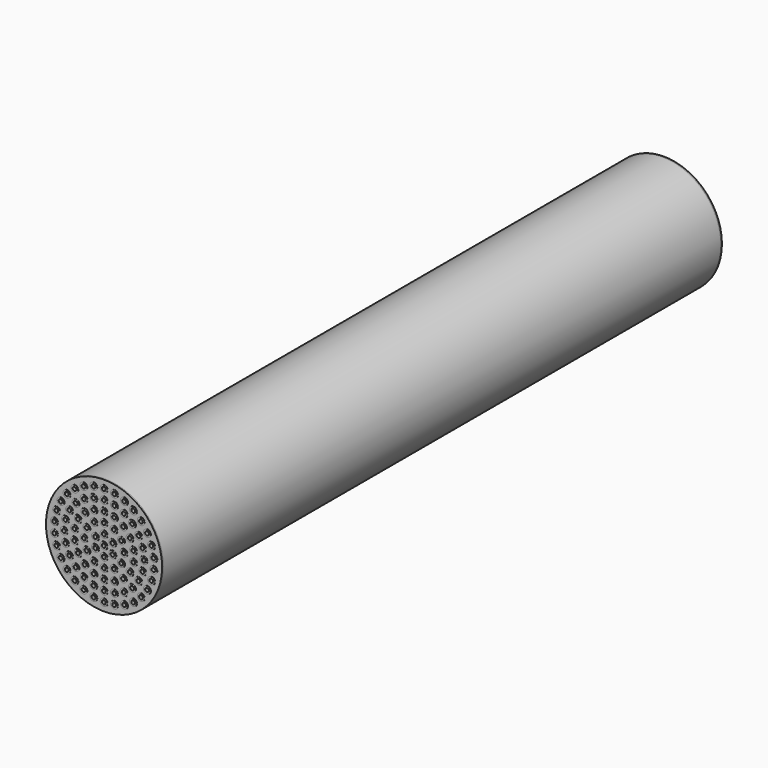
from build123d import *

# Parameters (mm, degrees)
F0_R          = 50.8
F0_R_2        = 49.276
F1_DEPTH      = 609.6
F0_R_3        = 3.175
F2_DEPTH      = 611.124
F2_DEPTH_BACK = 1.524
F3_T          = -1.524
F4_START      = 609.6
F4_DEPTH      = 1.27
F5_DEPTH      = 1.27


# Not quite as in the source:
# - a shell that OpenCascade refuses in one call is made with other operations: the cavity is built on its own and cut out


with BuildPart() as f1:
    # F0 (on Front) → F1 (new body)
    with BuildSketch(Plane.XZ):
        Circle(F0_R)
        Circle(F0_R_2, mode=Mode.SUBTRACT)
    extrude(amount=F1_DEPTH)


with BuildPart() as f2:
    # F0 (on Front) → F2 (new body, two sides)
    with BuildSketch(Plane.XZ) as f2_sk:
        with Locations((32.4429162872, 29.2117330339)):
            Circle(F0_R_3)
        with Locations((22.6844529204, -13.096875)):
            Circle(F0_R_3)
        with Locations((-9.0392551502, -33.7349594831)):
            Circle(F0_R_3)
        with Locations((-17.4625, -30.2459372272)):
            Circle(F0_R_3)
        with Locations((-8.9587901292, 24.6140735857)):
            Circle(F0_R_3)
        with Locations((-37.807421534, -21.828125)):
            Circle(F0_R_3)
        with Locations((-32.4429162872, -29.2117330339)):
            Circle(F0_R_3)
        with Locations((-30.2459372272, -17.4625)):
            Circle(F0_R_3)
        with Locations((-22.6844529204, 13.096875)):
            Circle(F0_R_3)
        with Locations((17.7565965743, -39.8819688852)):
            Circle(F0_R_3)
        with Locations((-9.0766447523, 42.7022561945)):
            Circle(F0_R_3)
        with Locations((25.7958080805, -4.5484969538)):
            Circle(F0_R_3)
        with Locations((0, -34.925)):
            Circle(F0_R_3)
        with Locations((-9.0766447523, -42.7022561945)):
            Circle(F0_R_3)
        with Locations((17.7565965743, 39.8819688852)):
            Circle(F0_R_3)
        with Locations((-25.6604999204, -35.3186481607)):
            Circle(F0_R_3)
        with Locations((-15.1229686136, -8.73125)):
            Circle(F0_R_3)
        with Locations((-41.5195610395, 13.4905231607)):
            Circle(F0_R_3)
        with Locations((9.0392551502, -33.7349594831)):
            Circle(F0_R_3)
        with Locations((-16.8370179512, -20.0655766319)):
            Circle(F0_R_3)
        with Locations((8.9587901292, -24.6140735857)):
            Circle(F0_R_3)
        with Locations((37.807421534, -21.828125)):
            Circle(F0_R_3)
        with Locations((16.8370179512, -20.0655766319)):
            Circle(F0_R_3)
        with Locations((25.7958080805, 4.5484969538)):
            Circle(F0_R_3)
        with Locations((43.4170964947, 4.5633207245)):
            Circle(F0_R_3)
        with Locations((-24.6957043329, -24.6957043329)):
            Circle(F0_R_3)
        with Locations((-33.7349594831, -9.0392551502)):
            Circle(F0_R_3)
        with Locations((-8.9587901292, -24.6140735857)):
            Circle(F0_R_3)
        with Locations((16.8370179512, 20.0655766319)):
            Circle(F0_R_3)
        with Locations((-15.1229686136, 8.73125)):
            Circle(F0_R_3)
        with Locations((33.7349594831, -9.0392551502)):
            Circle(F0_R_3)
        with Locations((9.0766447523, 42.7022561945)):
            Circle(F0_R_3)
        with Locations((0, 8.73125)):
            Circle(F0_R_3)
        with Locations((0, 34.925)):
            Circle(F0_R_3)
        with Locations((0, 43.65625)):
            Circle(F0_R_3)
        with Locations((-7.5614843068, -4.365625)):
            Circle(F0_R_3)
        with Locations((-7.5614843068, 4.365625)):
            Circle(F0_R_3)
        with Locations((7.5614843068, 4.365625)):
            Circle(F0_R_3)
        with Locations((-8.73125, 15.1229686136)):
            Circle(F0_R_3)
        with Locations((0, -17.4625)):
            Circle(F0_R_3)
        with Locations((37.807421534, 21.828125)):
            Circle(F0_R_3)
        with Locations((30.2459372272, -17.4625)):
            Circle(F0_R_3)
        with Locations((34.925, 0)):
            Circle(F0_R_3)
        with Locations((24.6957043329, 24.6957043329)):
            Circle(F0_R_3)
        with Locations((25.6604999204, 35.3186481607)):
            Circle(F0_R_3)
        with Locations((15.1229686136, -8.73125)):
            Circle(F0_R_3)
        with Locations((41.5195610395, -13.4905231607)):
            Circle(F0_R_3)
        with Locations((-37.807421534, 21.828125)):
            Circle(F0_R_3)
        with Locations((-43.4170964947, -4.5633207245)):
            Circle(F0_R_3)
        with Locations((41.5195610395, 13.4905231607)):
            Circle(F0_R_3)
        with Locations((17.4625, 0)):
            Circle(F0_R_3)
        with Locations((43.4170964947, -4.5633207245)):
            Circle(F0_R_3)
        with Locations((17.4625, 30.2459372272)):
            Circle(F0_R_3)
        with Locations((-34.925, 0)):
            Circle(F0_R_3)
        with Locations((-25.7958080805, -4.5484969538)):
            Circle(F0_R_3)
        with Locations((0, -26.19375)):
            Circle(F0_R_3)
        with Locations((15.1229686136, 8.73125)):
            Circle(F0_R_3)
        with Locations((-17.7565965743, -39.8819688852)):
            Circle(F0_R_3)
        with Locations((9.0766447523, -42.7022561945)):
            Circle(F0_R_3)
        with Locations((9.0392551502, 33.7349594831)):
            Circle(F0_R_3)
        with Locations((17.4625, -30.2459372272)):
            Circle(F0_R_3)
        with Locations((22.6844529204, 13.096875)):
            Circle(F0_R_3)
        with Locations((-22.6844529204, -13.096875)):
            Circle(F0_R_3)
        with Locations((-33.7349594831, 9.0392551502)):
            Circle(F0_R_3)
        with Locations((32.4429162872, -29.2117330339)):
            Circle(F0_R_3)
        with Locations((33.7349594831, 9.0392551502)):
            Circle(F0_R_3)
        with Locations((-17.4625, 30.2459372272)):
            Circle(F0_R_3)
        with Locations((-24.6957043329, 24.6957043329)):
            Circle(F0_R_3)
        with Locations((-25.7958080805, 4.5484969538)):
            Circle(F0_R_3)
        with Locations((24.6957043329, -24.6957043329)):
            Circle(F0_R_3)
        with Locations((8.73125, 15.1229686136)):
            Circle(F0_R_3)
        with Locations((-25.6604999204, 35.3186481607)):
            Circle(F0_R_3)
        with Locations((-17.4625, 0)):
            Circle(F0_R_3)
        with Locations((-8.73125, -15.1229686136)):
            Circle(F0_R_3)
        with Locations((25.6604999204, -35.3186481607)):
            Circle(F0_R_3)
        with Locations((-17.7565965743, 39.8819688852)):
            Circle(F0_R_3)
        with Locations((0, -43.65625)):
            Circle(F0_R_3)
        with Locations((30.2459372272, 17.4625)):
            Circle(F0_R_3)
        with Locations((-30.2459372272, 17.4625)):
            Circle(F0_R_3)
        with Locations((8.73125, -15.1229686136)):
            Circle(F0_R_3)
        Circle(F0_R_3)
        with Locations((-43.4170964947, 4.5633207245)):
            Circle(F0_R_3)
        with Locations((0, 26.19375)):
            Circle(F0_R_3)
        with Locations((0, 17.4625)):
            Circle(F0_R_3)
        with Locations((0, -8.73125)):
            Circle(F0_R_3)
        with Locations((-32.4429162872, 29.2117330339)):
            Circle(F0_R_3)
        with Locations((7.5614843068, -4.365625)):
            Circle(F0_R_3)
        with Locations((-9.0392551502, 33.7349594831)):
            Circle(F0_R_3)
        with Locations((8.9587901292, 24.6140735857)):
            Circle(F0_R_3)
        with Locations((-41.5195610395, -13.4905231607)):
            Circle(F0_R_3)
        with Locations((-16.8370179512, 20.0655766319)):
            Circle(F0_R_3)
    extrude(amount=F2_DEPTH)
    extrude(f2_sk.sketch, amount=-F2_DEPTH_BACK)

    # F3: a shell. OpenCascade refuses it in one call, so the cavity is built on its own and cut out:
    # the body offset inwards by the wall thickness, plus a prism from it out through each open face.
    f3_core = offset(f2.part, amount=F3_T, kind=Kind.INTERSECTION, mode=Mode.PRIVATE)
    f3_exits = [f3_core.faces().sort_by_distance(p)[0] for p in [
        (0, -609.6, -43.65625),
        (-9.076645, -609.6, -42.702256),
        (-17.756597, -609.6, -39.881969),
        (-25.6605, -609.6, -35.318648),
        (-32.442916, -609.6, -29.211733),
        (-37.807422, -609.6, -21.828125),
        (-41.519561, -609.6, -13.490523),
        (-43.417096, -609.6, -4.563321),
        (-43.417096, -609.6, 4.563321),
        (-41.519561, -609.6, 13.490523),
        (-37.807422, -609.6, 21.828125),
        (-32.442916, -609.6, 29.211733),
        (-25.6605, -609.6, 35.318648),
        (-17.756597, -609.6, 39.881969),
        (-9.076645, -609.6, 42.702256),
        (-30.245937, -609.6, -17.4625),
        (-33.734959, -609.6, -9.039255),
        (-34.925, -609.6, 0),
        (-33.734959, -609.6, 9.039255),
        (-30.245937, -609.6, 17.4625),
        (-24.695704, -609.6, 24.695704),
        (0, -609.6, 43.65625),
        (9.076645, -609.6, -42.702256),
        (-9.039255, -609.6, -33.734959),
        (-9.039255, -609.6, 33.734959),
        (17.756597, -609.6, 39.881969),
        (17.756597, -609.6, -39.881969),
        (0, -609.6, -34.925),
        (-17.4625, -609.6, -30.245937),
        (-24.695704, -609.6, -24.695704),
        (-17.4625, -609.6, 30.245937),
        (-16.837018, -609.6, -20.065577),
        (-22.684453, -609.6, -13.096875),
        (-25.795808, -609.6, -4.548497),
        (-25.795808, -609.6, 4.548497),
        (-22.684453, -609.6, 13.096875),
        (-16.837018, -609.6, 20.065577),
        (-8.95879, -609.6, 24.614074),
        (-15.122969, -609.6, -8.73125),
        (-17.4625, -609.6, 0),
        (-15.122969, -609.6, 8.73125),
        (0, -609.6, 34.925),
        (9.076645, -609.6, 42.702256),
        (9.039255, -609.6, 33.734959),
        (9.039255, -609.6, -33.734959),
        (-7.561484, -609.6, -4.365625),
        (-7.561484, -609.6, 4.365625),
        (25.6605, -609.6, 35.318648),
        (25.6605, -609.6, -35.318648),
        (17.4625, -609.6, 30.245937),
        (17.4625, -609.6, -30.245937),
        (8.95879, -609.6, 24.614074),
        (0, -609.6, -26.19375),
        (-8.95879, -609.6, -24.614074),
        (0, -609.6, -17.4625),
        (-8.73125, -609.6, -15.122969),
        (-8.73125, -609.6, 15.122969),
        (7.561484, -609.6, 4.365625),
        (7.561484, -609.6, -4.365625),
        (0, -609.6, -8.73125),
        (0, -609.6, 26.19375),
        (0, -609.6, 17.4625),
        (0, -609.6, 8.73125),
        (0, -609.6, 0),
        (32.442916, -609.6, 29.211733),
        (32.442916, -609.6, -29.211733),
        (24.695704, -609.6, 24.695704),
        (16.837018, -609.6, 20.065577),
        (25.795808, -609.6, 4.548497),
        (25.795808, -609.6, -4.548497),
        (16.837018, -609.6, -20.065577),
        (8.95879, -609.6, -24.614074),
        (8.73125, -609.6, 15.122969),
        (15.122969, -609.6, 8.73125),
        (17.4625, -609.6, 0),
        (15.122969, -609.6, -8.73125),
        (8.73125, -609.6, -15.122969),
        (37.807422, -609.6, 21.828125),
        (43.417096, -609.6, 4.563321),
        (43.417096, -609.6, -4.563321),
        (30.245937, -609.6, 17.4625),
        (33.734959, -609.6, 9.039255),
        (34.925, -609.6, 0),
        (33.734959, -609.6, -9.039255),
        (30.245937, -609.6, -17.4625),
        (24.695704, -609.6, -24.695704),
        (22.684453, -609.6, 13.096875),
        (22.684453, -609.6, -13.096875),
        (41.519561, -609.6, 13.490523),
        (41.519561, -609.6, -13.490523),
        (37.807422, -609.6, -21.828125),
        (-25.6605, 0, -35.318648),
        (-43.417096, 0, -4.563321),
        (0, 0, -43.65625),
        (-9.076645, 0, -42.702256),
        (-32.442916, 0, -29.211733),
        (-41.519561, 0, -13.490523),
        (-43.417096, 0, 4.563321),
        (-41.519561, 0, 13.490523),
        (-32.442916, 0, 29.211733),
        (-25.6605, 0, 35.318648),
        (-9.076645, 0, 42.702256),
        (0, 0, 43.65625),
        (-17.756597, 0, -39.881969),
        (-37.807422, 0, 21.828125),
        (-9.039255, 0, -33.734959),
        (-17.4625, 0, -30.245937),
        (-33.734959, 0, -9.039255),
        (-34.925, 0, 0),
        (-17.4625, 0, 30.245937),
        (17.756597, 0, -39.881969),
        (9.076645, 0, -42.702256),
        (-37.807422, 0, -21.828125),
        (-17.756597, 0, 39.881969),
        (17.4625, 0, 30.245937),
        (0, 0, -34.925),
        (-24.695704, 0, -24.695704),
        (-30.245937, 0, -17.4625),
        (-33.734959, 0, 9.039255),
        (-30.245937, 0, 17.4625),
        (-24.695704, 0, 24.695704),
        (-25.795808, 0, -4.548497),
        (9.076645, 0, 42.702256),
        (17.4625, 0, -30.245937),
        (9.039255, 0, -33.734959),
        (-9.039255, 0, 33.734959),
        (0, 0, -26.19375),
        (-22.684453, 0, -13.096875),
        (-25.795808, 0, 4.548497),
        (-16.837018, 0, 20.065577),
        (-15.122969, 0, -8.73125),
        (0, 0, 26.19375),
        (17.756597, 0, 39.881969),
        (25.6605, 0, -35.318648),
        (-8.95879, 0, -24.614074),
        (-16.837018, 0, -20.065577),
        (-22.684453, 0, 13.096875),
        (-8.95879, 0, 24.614074),
        (-8.73125, 0, -15.122969),
        (-17.4625, 0, 0),
        (-15.122969, 0, 8.73125),
        (0, 0, 34.925),
        (32.442916, 0, 29.211733),
        (32.442916, 0, -29.211733),
        (9.039255, 0, 33.734959),
        (8.95879, 0, 24.614074),
        (16.837018, 0, 20.065577),
        (8.95879, 0, -24.614074),
        (-8.73125, 0, 15.122969),
        (0, 0, -8.73125),
        (-7.561484, 0, -4.365625),
        (-7.561484, 0, 4.365625),
        (0, 0, 17.4625),
        (25.6605, 0, 35.318648),
        (24.695704, 0, -24.695704),
        (8.73125, 0, -15.122969),
        (0, 0, -17.4625),
        (7.561484, 0, 4.365625),
        (0, 0, 8.73125),
        (37.807422, 0, 21.828125),
        (24.695704, 0, 24.695704),
        (30.245937, 0, 17.4625),
        (22.684453, 0, -13.096875),
        (16.837018, 0, -20.065577),
        (8.73125, 0, 15.122969),
        (15.122969, 0, -8.73125),
        (7.561484, 0, -4.365625),
        (0, 0, 0),
        (41.519561, 0, -13.490523),
        (37.807422, 0, -21.828125),
        (25.795808, 0, 4.548497),
        (25.795808, 0, -4.548497),
        (15.122969, 0, 8.73125),
        (41.519561, 0, 13.490523),
        (33.734959, 0, 9.039255),
        (33.734959, 0, -9.039255),
        (30.245937, 0, -17.4625),
        (22.684453, 0, 13.096875),
        (17.4625, 0, 0),
        (43.417096, 0, 4.563321),
        (43.417096, 0, -4.563321),
        (34.925, 0, 0),
    ]]
    add(f3_core, mode=Mode.SUBTRACT)
    extrude(f3_exits, amount=-F3_T, mode=Mode.SUBTRACT)


with BuildPart() as f4:
    # F0 (on Front) → F4 (new body)
    with BuildSketch(Plane.XZ.offset(F4_START)):
        Circle(F0_R)
        Circle(F0_R_2, mode=Mode.SUBTRACT)
        Circle(F0_R_2)
        with Locations((-25.6604999204, -35.3186481607)):
            Circle(F0_R_3, mode=Mode.SUBTRACT)
        with Locations((-32.4429162872, -29.2117330339)):
            Circle(F0_R_3, mode=Mode.SUBTRACT)
        with Locations((-17.7565965743, -39.8819688852)):
            Circle(F0_R_3, mode=Mode.SUBTRACT)
        with Locations((-9.0766447523, -42.7022561945)):
            Circle(F0_R_3, mode=Mode.SUBTRACT)
        with Locations((0, -43.65625)):
            Circle(F0_R_3, mode=Mode.SUBTRACT)
        with Locations((-17.4625, -30.2459372272)):
            Circle(F0_R_3, mode=Mode.SUBTRACT)
        with Locations((-9.0392551502, -33.7349594831)):
            Circle(F0_R_3, mode=Mode.SUBTRACT)
        with Locations((0, -34.925)):
            Circle(F0_R_3, mode=Mode.SUBTRACT)
        with Locations((0, -26.19375)):
            Circle(F0_R_3, mode=Mode.SUBTRACT)
        with Locations((-41.5195610395, -13.4905231607)):
            Circle(F0_R_3, mode=Mode.SUBTRACT)
        with Locations((-37.807421534, -21.828125)):
            Circle(F0_R_3, mode=Mode.SUBTRACT)
        with Locations((-30.2459372272, -17.4625)):
            Circle(F0_R_3, mode=Mode.SUBTRACT)
        with Locations((-43.4170964947, -4.5633207245)):
            Circle(F0_R_3, mode=Mode.SUBTRACT)
        with Locations((-33.7349594831, -9.0392551502)):
            Circle(F0_R_3, mode=Mode.SUBTRACT)
        with Locations((-34.925, 0)):
            Circle(F0_R_3, mode=Mode.SUBTRACT)
        with Locations((-25.7958080805, -4.5484969538)):
            Circle(F0_R_3, mode=Mode.SUBTRACT)
        with Locations((-24.6957043329, -24.6957043329)):
            Circle(F0_R_3, mode=Mode.SUBTRACT)
        with Locations((-16.8370179512, -20.0655766319)):
            Circle(F0_R_3, mode=Mode.SUBTRACT)
        with Locations((-22.6844529204, -13.096875)):
            Circle(F0_R_3, mode=Mode.SUBTRACT)
        with Locations((-8.9587901292, -24.6140735857)):
            Circle(F0_R_3, mode=Mode.SUBTRACT)
        with Locations((-8.73125, -15.1229686136)):
            Circle(F0_R_3, mode=Mode.SUBTRACT)
        with Locations((0, -17.4625)):
            Circle(F0_R_3, mode=Mode.SUBTRACT)
        with Locations((-15.1229686136, -8.73125)):
            Circle(F0_R_3, mode=Mode.SUBTRACT)
        with Locations((-17.4625, 0)):
            Circle(F0_R_3, mode=Mode.SUBTRACT)
        with Locations((0, -8.73125)):
            Circle(F0_R_3, mode=Mode.SUBTRACT)
        with Locations((-7.5614843068, -4.365625)):
            Circle(F0_R_3, mode=Mode.SUBTRACT)
        Circle(F0_R_3, mode=Mode.SUBTRACT)
        with Locations((9.0766447523, -42.7022561945)):
            Circle(F0_R_3, mode=Mode.SUBTRACT)
        with Locations((17.7565965743, -39.8819688852)):
            Circle(F0_R_3, mode=Mode.SUBTRACT)
        with Locations((9.0392551502, -33.7349594831)):
            Circle(F0_R_3, mode=Mode.SUBTRACT)
        with Locations((17.4625, -30.2459372272)):
            Circle(F0_R_3, mode=Mode.SUBTRACT)
        with Locations((25.6604999204, -35.3186481607)):
            Circle(F0_R_3, mode=Mode.SUBTRACT)
        with Locations((32.4429162872, -29.2117330339)):
            Circle(F0_R_3, mode=Mode.SUBTRACT)
        with Locations((8.9587901292, -24.6140735857)):
            Circle(F0_R_3, mode=Mode.SUBTRACT)
        with Locations((8.73125, -15.1229686136)):
            Circle(F0_R_3, mode=Mode.SUBTRACT)
        with Locations((16.8370179512, -20.0655766319)):
            Circle(F0_R_3, mode=Mode.SUBTRACT)
        with Locations((24.6957043329, -24.6957043329)):
            Circle(F0_R_3, mode=Mode.SUBTRACT)
        with Locations((22.6844529204, -13.096875)):
            Circle(F0_R_3, mode=Mode.SUBTRACT)
        with Locations((7.5614843068, -4.365625)):
            Circle(F0_R_3, mode=Mode.SUBTRACT)
        with Locations((15.1229686136, -8.73125)):
            Circle(F0_R_3, mode=Mode.SUBTRACT)
        with Locations((17.4625, 0)):
            Circle(F0_R_3, mode=Mode.SUBTRACT)
        with Locations((37.807421534, -21.828125)):
            Circle(F0_R_3, mode=Mode.SUBTRACT)
        with Locations((30.2459372272, -17.4625)):
            Circle(F0_R_3, mode=Mode.SUBTRACT)
        with Locations((41.5195610395, -13.4905231607)):
            Circle(F0_R_3, mode=Mode.SUBTRACT)
        with Locations((33.7349594831, -9.0392551502)):
            Circle(F0_R_3, mode=Mode.SUBTRACT)
        with Locations((25.7958080805, -4.5484969538)):
            Circle(F0_R_3, mode=Mode.SUBTRACT)
        with Locations((34.925, 0)):
            Circle(F0_R_3, mode=Mode.SUBTRACT)
        with Locations((43.4170964947, -4.5633207245)):
            Circle(F0_R_3, mode=Mode.SUBTRACT)
        with Locations((-43.4170964947, 4.5633207245)):
            Circle(F0_R_3, mode=Mode.SUBTRACT)
        with Locations((-25.7958080805, 4.5484969538)):
            Circle(F0_R_3, mode=Mode.SUBTRACT)
        with Locations((-33.7349594831, 9.0392551502)):
            Circle(F0_R_3, mode=Mode.SUBTRACT)
        with Locations((-41.5195610395, 13.4905231607)):
            Circle(F0_R_3, mode=Mode.SUBTRACT)
        with Locations((-30.2459372272, 17.4625)):
            Circle(F0_R_3, mode=Mode.SUBTRACT)
        with Locations((-37.807421534, 21.828125)):
            Circle(F0_R_3, mode=Mode.SUBTRACT)
        with Locations((-15.1229686136, 8.73125)):
            Circle(F0_R_3, mode=Mode.SUBTRACT)
        with Locations((-7.5614843068, 4.365625)):
            Circle(F0_R_3, mode=Mode.SUBTRACT)
        with Locations((0, 8.73125)):
            Circle(F0_R_3, mode=Mode.SUBTRACT)
        with Locations((-22.6844529204, 13.096875)):
            Circle(F0_R_3, mode=Mode.SUBTRACT)
        with Locations((-24.6957043329, 24.6957043329)):
            Circle(F0_R_3, mode=Mode.SUBTRACT)
        with Locations((-16.8370179512, 20.0655766319)):
            Circle(F0_R_3, mode=Mode.SUBTRACT)
        with Locations((-8.73125, 15.1229686136)):
            Circle(F0_R_3, mode=Mode.SUBTRACT)
        with Locations((0, 17.4625)):
            Circle(F0_R_3, mode=Mode.SUBTRACT)
        with Locations((-8.9587901292, 24.6140735857)):
            Circle(F0_R_3, mode=Mode.SUBTRACT)
        with Locations((-32.4429162872, 29.2117330339)):
            Circle(F0_R_3, mode=Mode.SUBTRACT)
        with Locations((-25.6604999204, 35.3186481607)):
            Circle(F0_R_3, mode=Mode.SUBTRACT)
        with Locations((-17.4625, 30.2459372272)):
            Circle(F0_R_3, mode=Mode.SUBTRACT)
        with Locations((0, 26.19375)):
            Circle(F0_R_3, mode=Mode.SUBTRACT)
        with Locations((-9.0392551502, 33.7349594831)):
            Circle(F0_R_3, mode=Mode.SUBTRACT)
        with Locations((0, 34.925)):
            Circle(F0_R_3, mode=Mode.SUBTRACT)
        with Locations((-17.7565965743, 39.8819688852)):
            Circle(F0_R_3, mode=Mode.SUBTRACT)
        with Locations((-9.0766447523, 42.7022561945)):
            Circle(F0_R_3, mode=Mode.SUBTRACT)
        with Locations((0, 43.65625)):
            Circle(F0_R_3, mode=Mode.SUBTRACT)
        with Locations((7.5614843068, 4.365625)):
            Circle(F0_R_3, mode=Mode.SUBTRACT)
        with Locations((15.1229686136, 8.73125)):
            Circle(F0_R_3, mode=Mode.SUBTRACT)
        with Locations((8.73125, 15.1229686136)):
            Circle(F0_R_3, mode=Mode.SUBTRACT)
        with Locations((8.9587901292, 24.6140735857)):
            Circle(F0_R_3, mode=Mode.SUBTRACT)
        with Locations((22.6844529204, 13.096875)):
            Circle(F0_R_3, mode=Mode.SUBTRACT)
        with Locations((16.8370179512, 20.0655766319)):
            Circle(F0_R_3, mode=Mode.SUBTRACT)
        with Locations((24.6957043329, 24.6957043329)):
            Circle(F0_R_3, mode=Mode.SUBTRACT)
        with Locations((25.7958080805, 4.5484969538)):
            Circle(F0_R_3, mode=Mode.SUBTRACT)
        with Locations((33.7349594831, 9.0392551502)):
            Circle(F0_R_3, mode=Mode.SUBTRACT)
        with Locations((43.4170964947, 4.5633207245)):
            Circle(F0_R_3, mode=Mode.SUBTRACT)
        with Locations((30.2459372272, 17.4625)):
            Circle(F0_R_3, mode=Mode.SUBTRACT)
        with Locations((37.807421534, 21.828125)):
            Circle(F0_R_3, mode=Mode.SUBTRACT)
        with Locations((41.5195610395, 13.4905231607)):
            Circle(F0_R_3, mode=Mode.SUBTRACT)
        with Locations((9.0392551502, 33.7349594831)):
            Circle(F0_R_3, mode=Mode.SUBTRACT)
        with Locations((17.4625, 30.2459372272)):
            Circle(F0_R_3, mode=Mode.SUBTRACT)
        with Locations((9.0766447523, 42.7022561945)):
            Circle(F0_R_3, mode=Mode.SUBTRACT)
        with Locations((17.7565965743, 39.8819688852)):
            Circle(F0_R_3, mode=Mode.SUBTRACT)
        with Locations((32.4429162872, 29.2117330339)):
            Circle(F0_R_3, mode=Mode.SUBTRACT)
        with Locations((25.6604999204, 35.3186481607)):
            Circle(F0_R_3, mode=Mode.SUBTRACT)
    extrude(amount=F4_DEPTH)


with BuildPart() as f5:
    # F0 (on Front) → F5 (new body)
    with BuildSketch(Plane.XZ):
        Circle(F0_R)
        Circle(F0_R_2, mode=Mode.SUBTRACT)
        Circle(F0_R_2)
        with Locations((-25.6604999204, -35.3186481607)):
            Circle(F0_R_3, mode=Mode.SUBTRACT)
        with Locations((-32.4429162872, -29.2117330339)):
            Circle(F0_R_3, mode=Mode.SUBTRACT)
        with Locations((-17.7565965743, -39.8819688852)):
            Circle(F0_R_3, mode=Mode.SUBTRACT)
        with Locations((-9.0766447523, -42.7022561945)):
            Circle(F0_R_3, mode=Mode.SUBTRACT)
        with Locations((0, -43.65625)):
            Circle(F0_R_3, mode=Mode.SUBTRACT)
        with Locations((-17.4625, -30.2459372272)):
            Circle(F0_R_3, mode=Mode.SUBTRACT)
        with Locations((-9.0392551502, -33.7349594831)):
            Circle(F0_R_3, mode=Mode.SUBTRACT)
        with Locations((0, -34.925)):
            Circle(F0_R_3, mode=Mode.SUBTRACT)
        with Locations((0, -26.19375)):
            Circle(F0_R_3, mode=Mode.SUBTRACT)
        with Locations((-41.5195610395, -13.4905231607)):
            Circle(F0_R_3, mode=Mode.SUBTRACT)
        with Locations((-37.807421534, -21.828125)):
            Circle(F0_R_3, mode=Mode.SUBTRACT)
        with Locations((-30.2459372272, -17.4625)):
            Circle(F0_R_3, mode=Mode.SUBTRACT)
        with Locations((-43.4170964947, -4.5633207245)):
            Circle(F0_R_3, mode=Mode.SUBTRACT)
        with Locations((-33.7349594831, -9.0392551502)):
            Circle(F0_R_3, mode=Mode.SUBTRACT)
        with Locations((-34.925, 0)):
            Circle(F0_R_3, mode=Mode.SUBTRACT)
        with Locations((-25.7958080805, -4.5484969538)):
            Circle(F0_R_3, mode=Mode.SUBTRACT)
        with Locations((-24.6957043329, -24.6957043329)):
            Circle(F0_R_3, mode=Mode.SUBTRACT)
        with Locations((-16.8370179512, -20.0655766319)):
            Circle(F0_R_3, mode=Mode.SUBTRACT)
        with Locations((-22.6844529204, -13.096875)):
            Circle(F0_R_3, mode=Mode.SUBTRACT)
        with Locations((-8.9587901292, -24.6140735857)):
            Circle(F0_R_3, mode=Mode.SUBTRACT)
        with Locations((-8.73125, -15.1229686136)):
            Circle(F0_R_3, mode=Mode.SUBTRACT)
        with Locations((0, -17.4625)):
            Circle(F0_R_3, mode=Mode.SUBTRACT)
        with Locations((-15.1229686136, -8.73125)):
            Circle(F0_R_3, mode=Mode.SUBTRACT)
        with Locations((-17.4625, 0)):
            Circle(F0_R_3, mode=Mode.SUBTRACT)
        with Locations((0, -8.73125)):
            Circle(F0_R_3, mode=Mode.SUBTRACT)
        with Locations((-7.5614843068, -4.365625)):
            Circle(F0_R_3, mode=Mode.SUBTRACT)
        Circle(F0_R_3, mode=Mode.SUBTRACT)
        with Locations((9.0766447523, -42.7022561945)):
            Circle(F0_R_3, mode=Mode.SUBTRACT)
        with Locations((17.7565965743, -39.8819688852)):
            Circle(F0_R_3, mode=Mode.SUBTRACT)
        with Locations((9.0392551502, -33.7349594831)):
            Circle(F0_R_3, mode=Mode.SUBTRACT)
        with Locations((17.4625, -30.2459372272)):
            Circle(F0_R_3, mode=Mode.SUBTRACT)
        with Locations((25.6604999204, -35.3186481607)):
            Circle(F0_R_3, mode=Mode.SUBTRACT)
        with Locations((32.4429162872, -29.2117330339)):
            Circle(F0_R_3, mode=Mode.SUBTRACT)
        with Locations((8.9587901292, -24.6140735857)):
            Circle(F0_R_3, mode=Mode.SUBTRACT)
        with Locations((8.73125, -15.1229686136)):
            Circle(F0_R_3, mode=Mode.SUBTRACT)
        with Locations((16.8370179512, -20.0655766319)):
            Circle(F0_R_3, mode=Mode.SUBTRACT)
        with Locations((24.6957043329, -24.6957043329)):
            Circle(F0_R_3, mode=Mode.SUBTRACT)
        with Locations((22.6844529204, -13.096875)):
            Circle(F0_R_3, mode=Mode.SUBTRACT)
        with Locations((7.5614843068, -4.365625)):
            Circle(F0_R_3, mode=Mode.SUBTRACT)
        with Locations((15.1229686136, -8.73125)):
            Circle(F0_R_3, mode=Mode.SUBTRACT)
        with Locations((17.4625, 0)):
            Circle(F0_R_3, mode=Mode.SUBTRACT)
        with Locations((37.807421534, -21.828125)):
            Circle(F0_R_3, mode=Mode.SUBTRACT)
        with Locations((30.2459372272, -17.4625)):
            Circle(F0_R_3, mode=Mode.SUBTRACT)
        with Locations((41.5195610395, -13.4905231607)):
            Circle(F0_R_3, mode=Mode.SUBTRACT)
        with Locations((33.7349594831, -9.0392551502)):
            Circle(F0_R_3, mode=Mode.SUBTRACT)
        with Locations((25.7958080805, -4.5484969538)):
            Circle(F0_R_3, mode=Mode.SUBTRACT)
        with Locations((34.925, 0)):
            Circle(F0_R_3, mode=Mode.SUBTRACT)
        with Locations((43.4170964947, -4.5633207245)):
            Circle(F0_R_3, mode=Mode.SUBTRACT)
        with Locations((-43.4170964947, 4.5633207245)):
            Circle(F0_R_3, mode=Mode.SUBTRACT)
        with Locations((-25.7958080805, 4.5484969538)):
            Circle(F0_R_3, mode=Mode.SUBTRACT)
        with Locations((-33.7349594831, 9.0392551502)):
            Circle(F0_R_3, mode=Mode.SUBTRACT)
        with Locations((-41.5195610395, 13.4905231607)):
            Circle(F0_R_3, mode=Mode.SUBTRACT)
        with Locations((-30.2459372272, 17.4625)):
            Circle(F0_R_3, mode=Mode.SUBTRACT)
        with Locations((-37.807421534, 21.828125)):
            Circle(F0_R_3, mode=Mode.SUBTRACT)
        with Locations((-15.1229686136, 8.73125)):
            Circle(F0_R_3, mode=Mode.SUBTRACT)
        with Locations((-7.5614843068, 4.365625)):
            Circle(F0_R_3, mode=Mode.SUBTRACT)
        with Locations((0, 8.73125)):
            Circle(F0_R_3, mode=Mode.SUBTRACT)
        with Locations((-22.6844529204, 13.096875)):
            Circle(F0_R_3, mode=Mode.SUBTRACT)
        with Locations((-24.6957043329, 24.6957043329)):
            Circle(F0_R_3, mode=Mode.SUBTRACT)
        with Locations((-16.8370179512, 20.0655766319)):
            Circle(F0_R_3, mode=Mode.SUBTRACT)
        with Locations((-8.73125, 15.1229686136)):
            Circle(F0_R_3, mode=Mode.SUBTRACT)
        with Locations((0, 17.4625)):
            Circle(F0_R_3, mode=Mode.SUBTRACT)
        with Locations((-8.9587901292, 24.6140735857)):
            Circle(F0_R_3, mode=Mode.SUBTRACT)
        with Locations((-32.4429162872, 29.2117330339)):
            Circle(F0_R_3, mode=Mode.SUBTRACT)
        with Locations((-25.6604999204, 35.3186481607)):
            Circle(F0_R_3, mode=Mode.SUBTRACT)
        with Locations((-17.4625, 30.2459372272)):
            Circle(F0_R_3, mode=Mode.SUBTRACT)
        with Locations((0, 26.19375)):
            Circle(F0_R_3, mode=Mode.SUBTRACT)
        with Locations((-9.0392551502, 33.7349594831)):
            Circle(F0_R_3, mode=Mode.SUBTRACT)
        with Locations((0, 34.925)):
            Circle(F0_R_3, mode=Mode.SUBTRACT)
        with Locations((-17.7565965743, 39.8819688852)):
            Circle(F0_R_3, mode=Mode.SUBTRACT)
        with Locations((-9.0766447523, 42.7022561945)):
            Circle(F0_R_3, mode=Mode.SUBTRACT)
        with Locations((0, 43.65625)):
            Circle(F0_R_3, mode=Mode.SUBTRACT)
        with Locations((7.5614843068, 4.365625)):
            Circle(F0_R_3, mode=Mode.SUBTRACT)
        with Locations((15.1229686136, 8.73125)):
            Circle(F0_R_3, mode=Mode.SUBTRACT)
        with Locations((8.73125, 15.1229686136)):
            Circle(F0_R_3, mode=Mode.SUBTRACT)
        with Locations((8.9587901292, 24.6140735857)):
            Circle(F0_R_3, mode=Mode.SUBTRACT)
        with Locations((22.6844529204, 13.096875)):
            Circle(F0_R_3, mode=Mode.SUBTRACT)
        with Locations((16.8370179512, 20.0655766319)):
            Circle(F0_R_3, mode=Mode.SUBTRACT)
        with Locations((24.6957043329, 24.6957043329)):
            Circle(F0_R_3, mode=Mode.SUBTRACT)
        with Locations((25.7958080805, 4.5484969538)):
            Circle(F0_R_3, mode=Mode.SUBTRACT)
        with Locations((33.7349594831, 9.0392551502)):
            Circle(F0_R_3, mode=Mode.SUBTRACT)
        with Locations((43.4170964947, 4.5633207245)):
            Circle(F0_R_3, mode=Mode.SUBTRACT)
        with Locations((30.2459372272, 17.4625)):
            Circle(F0_R_3, mode=Mode.SUBTRACT)
        with Locations((37.807421534, 21.828125)):
            Circle(F0_R_3, mode=Mode.SUBTRACT)
        with Locations((41.5195610395, 13.4905231607)):
            Circle(F0_R_3, mode=Mode.SUBTRACT)
        with Locations((9.0392551502, 33.7349594831)):
            Circle(F0_R_3, mode=Mode.SUBTRACT)
        with Locations((17.4625, 30.2459372272)):
            Circle(F0_R_3, mode=Mode.SUBTRACT)
        with Locations((9.0766447523, 42.7022561945)):
            Circle(F0_R_3, mode=Mode.SUBTRACT)
        with Locations((17.7565965743, 39.8819688852)):
            Circle(F0_R_3, mode=Mode.SUBTRACT)
        with Locations((32.4429162872, 29.2117330339)):
            Circle(F0_R_3, mode=Mode.SUBTRACT)
        with Locations((25.6604999204, 35.3186481607)):
            Circle(F0_R_3, mode=Mode.SUBTRACT)
    extrude(amount=-F5_DEPTH)


solid = Compound([f1.part, f2.part, f4.part, f5.part])
